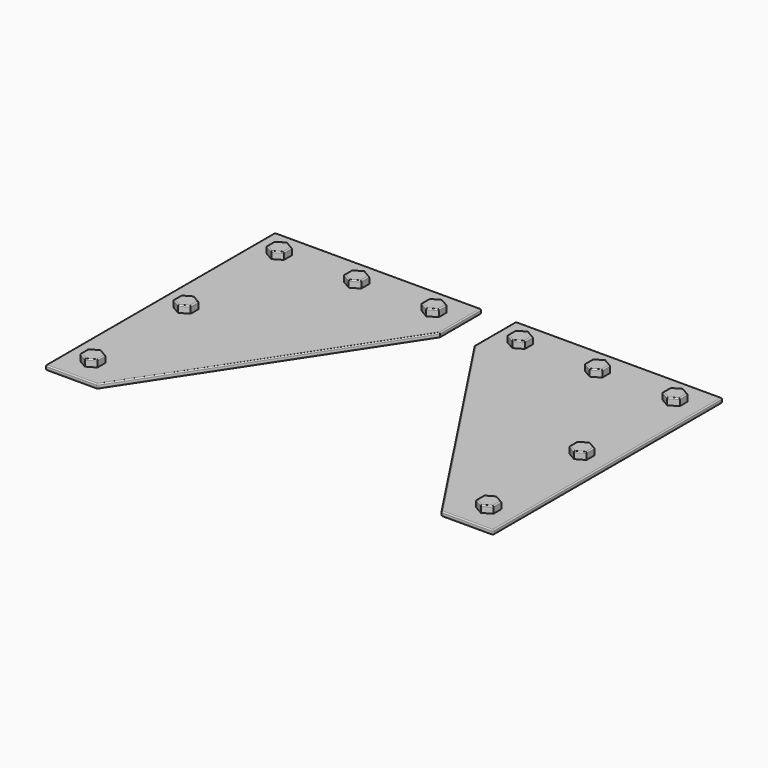
from build123d import *

# Parameters (mm, degrees)
F1_DEPTH = 4
F2_R     = 1
F4_DEPTH = 6
F5_R     = 1


with BuildPart() as f1:
    # F0 (on Top) → F1 (new body)
    with BuildSketch(Plane.XY):
        Polygon((195, 200), (15, 200), (15, 155), (150, -50), (195, -50), align=None)
    extrude(amount=F1_DEPTH)

    # F2
    f2_edges = [f1.edges().sort_by_distance(p)[0] for p in [
        (105, 200, 4),
        (15, 177.5, 4),
        (82.5, 52.5, 4),
        (172.5, -50, 4),
        (195, 75, 4),
        (105, 200, 0),
        (15, 177.5, 0),
        (82.5, 52.5, 0),
        (172.5, -50, 0),
        (195, 75, 0),
        (195, -50, 2),
        (195, 200, 2),
        (15, 200, 2),
        (150, -50, 2),
    ]]
    fillet(f2_edges, radius=F2_R)

    # F3 (on face) → F4 (join)
    with BuildSketch(Plane.XY.offset(4)):
        Polygon((37.5, 167.8397459622), (45, 172.1698729811), (45, 180.8301270189), (37.5, 185.1602540378), (30, 180.8301270189), (30, 172.1698729811), align=None)
        Polygon((112.5, 180.8301270189), (105, 185.1602540378), (97.5, 180.8301270189), (97.5, 172.1698729811), (105, 167.8397459622), (112.5, 172.1698729811), align=None)
        Polygon((180, 180.8301270189), (172.5, 185.1602540378), (165, 180.8301270189), (165, 172.1698729811), (172.5, 167.8397459622), (180, 172.1698729811), align=None)
        Polygon((165, 79.3301270189), (165, 70.6698729811), (172.5, 66.3397459622), (180, 70.6698729811), (180, 79.3301270189), (172.5, 83.6602540378), align=None)
        Polygon((165, -22.1698729811), (165, -30.8301270189), (172.5, -35.1602540378), (180, -30.8301270189), (180, -22.1698729811), (172.5, -17.8397459622), align=None)
    extrude(amount=F4_DEPTH)

    # F5
    f5_edges = [f1.edges().sort_by_distance(p)[0] for p in [
        (165, -26.5, 10),
        (168.75, -32.995191, 10),
        (176.25, -32.995191, 10),
        (180, -26.5, 10),
        (176.25, -20.004809, 10),
        (168.75, -20.004809, 10),
        (165, 75, 10),
        (168.75, 68.504809, 10),
        (176.25, 68.504809, 10),
        (180, 75, 10),
        (176.25, 81.495191, 10),
        (168.75, 81.495191, 10),
        (176.25, 170.004809, 10),
        (180, 176.5, 10),
        (176.25, 182.995191, 10),
        (168.75, 182.995191, 10),
        (165, 176.5, 10),
        (168.75, 170.004809, 10),
        (108.75, 182.995191, 10),
        (101.25, 182.995191, 10),
        (97.5, 176.5, 10),
        (101.25, 170.004809, 10),
        (108.75, 170.004809, 10),
        (112.5, 176.5, 10),
        (41.25, 170.004809, 10),
        (45, 176.5, 10),
        (41.25, 182.995191, 10),
        (33.75, 182.995191, 10),
        (30, 176.5, 10),
        (33.75, 170.004809, 10),
    ]]
    fillet(f5_edges, radius=F5_R)


with BuildPart() as f6_1:
    # F6: instance of F1
    add(f1.part.mirror(Plane.YZ))


solid = Compound([f1.part, f6_1.part])
